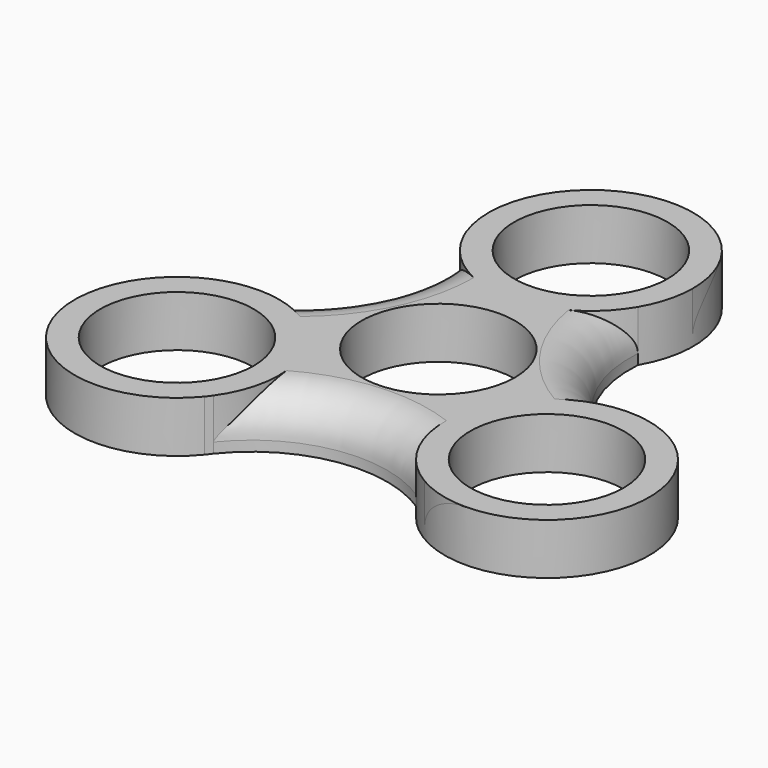
from build123d import *

# Parameters (mm, degrees)
F0_R         = 9.525
F1_DEPTH     = 6.35
F2_T4_ANGLE  = 171.8918539933
F2_S5_R      = 12.7
F2_T6_DEPTH  = 33
F2_S7_R      = 12.7
F2_T8_DEPTH  = 33
F2_T12_ANGLE = 171.8918539933
F2_S13_R     = 12.7
F2_T14_DEPTH = 34
F2_S15_R     = 12.7
F2_T16_DEPTH = 34
F2_T20_ANGLE = 171.8918539933
F2_S21_R     = 12.7
F2_T22_DEPTH = 33
F2_S23_R     = 12.7
F2_T24_DEPTH = 33


# Not quite as in the source:
# - a fillet or chamfer that OpenCascade refuses, or shapes differently, is made with other operations: its cross-section is extruded or revolved along the edge and cut away or added


with BuildPart() as f1:
    # F0 (on Top) → F1 (new body)
    with BuildSketch(Plane.XY):
        with BuildLine():
            ThreePointArc((-16.9151689036, 34.8937534074), (-16.926787396, 22.6379285555), (-25.2467054302, 13.6387985033))
            ThreePointArc((-25.2467054302, 13.6387985033), (-36.7990792752, -4.4780457484), (-15.4716495202, -7.0892001179))
            ThreePointArc((-15.4716495202, -7.0892001179), (-15.2019637006, -6.723178945), (-14.922490674, -6.3645750302))
            ThreePointArc((-14.922490674, -6.3645750302), (-4.3028257617, -0.2467245138), (7.6506084925, -2.9524198627))
            ThreePointArc((7.6506084925, -2.9524198627), (29.1164427734, -3.8986469606), (20.7140539132, 15.8770261894))
            ThreePointArc((20.7140539132, 15.8770261894), (20.2622273693, 15.9275703737), (19.8119307558, 15.9902991571))
            ThreePointArc((19.8119307558, 15.9902991571), (9.2038843359, 22.1282734926), (5.5703681159, 33.8330988937))
            ThreePointArc((5.5703681159, 33.8330988937), (-4.34309232, 52.8961702433), (-17.2681332147, 35.7316514628))
            ThreePointArc((-17.2681332147, 35.7316514628), (-17.0859924904, 35.3150861055), (-16.9151689036, 34.8937534074))
        make_face()
        with Locations((-25.31230589, 0.9389679304)):
            Circle(F0_R, mode=Mode.SUBTRACT)
        with Locations((-4.0085762739, 14.8398258448)):
            Circle(F0_R, mode=Mode.SUBTRACT)
        with Locations((18.6817846223, 3.3406837591)):
            Circle(F0_R, mode=Mode.SUBTRACT)
        with Locations((-5.3952075541, 40.2398258448)):
            Circle(F0_R, mode=Mode.SUBTRACT)
        with BuildLine():
            ThreePointArc((-14.922490674, -6.3645750302), (-15.2019637006, -6.723178945), (-15.4716495202, -7.0892001179))
            ThreePointArc((-15.4716495202, -7.0892001179), (-15.1905834316, -6.7318035089), (-14.922490674, -6.3645750302))
        make_face()
        with BuildLine():
            ThreePointArc((-17.2681332147, 35.7316514628), (-17.0991517164, 35.3095427854), (-16.9151689036, 34.8937534074))
            ThreePointArc((-16.9151689036, 34.8937534074), (-17.0859924904, 35.3150861055), (-17.2681332147, 35.7316514628))
        make_face()
        with BuildLine():
            ThreePointArc((19.8119307558, 15.9902991571), (20.2622273693, 15.9275703737), (20.7140539132, 15.8770261894))
            ThreePointArc((20.7140539132, 15.8770261894), (20.2640063262, 15.9417382578), (19.8119307558, 15.9902991571))
        make_face()
    extrude(amount=F1_DEPTH)

    # F2: fillet of radius 5.08 on 3 edges, made by hand


with BuildPart() as f2_tool2:
    # F2_s3 → F2_t4 (revolve)
    with BuildSketch(Plane(origin=(1.3219976545, -16.6427211425, 0), x_dir=(0, 0, 1), z_dir=(0.0791845597, -0.9968599729, 0))):
        with BuildLine():
            ThreePointArc((1.27, 19.9508919573), (4.8621024484, 21.4387895089), (6.35, 25.0308919573))
            Line((6.35, 25.0308919573), (6.35, 19.9508919573))
            Line((6.35, 19.9508919573), (1.27, 19.9508919573))
        make_face()
    revolve(axis=Axis((-1.7870715149, -16.8896868949, 6.35), (0, 0, -1)), revolution_arc=F2_T4_ANGLE)

    # F2_s5 → F2_t6 (cut, symmetric)
    with BuildSketch(Plane.XY.offset(2)):
        with Locations((-25.31230589, 0.9389679304)):
            Circle(F2_S5_R)
    extrude(amount=F2_T6_DEPTH, both=True, mode=Mode.SUBTRACT)

    # F2_s7 → F2_t8 (cut, symmetric)
    with BuildSketch(Plane.XY.offset(2)):
        with Locations((18.6817846223, 3.3406837591)):
            Circle(F2_S7_R)
    extrude(amount=F2_T8_DEPTH, both=True, mode=Mode.SUBTRACT)


with BuildPart() as f1_1:
    add(f1.part)

    # F2_t1: cut F2_tool2
    add(f2_tool2.part, mode=Mode.SUBTRACT)


with BuildPart() as f2_tool10:
    # F2_s11 → F2_t12 (revolve)
    with BuildSketch(Plane(origin=(30.4099792651, 20.9327995218, 0), x_dir=(0, 0, 1), z_dir=(0.8237137807, 0.5670058267, 0))):
        with BuildLine():
            ThreePointArc((1.27, 2.6333326422), (4.8621024484, 4.1212301938), (6.35, 7.7133326422))
            Line((6.35, 7.7133326422), (6.35, 2.6333326422))
            Line((6.35, 2.6333326422), (1.27, 2.6333326422))
        make_face()
    revolve(axis=Axis((22.3592354288, 32.6284617706, 6.35), (0, 0, -1)), revolution_arc=F2_T12_ANGLE)

    # F2_s13 → F2_t14 (cut, symmetric)
    with BuildSketch(Plane.XY.offset(2)):
        with Locations((18.6817846223, 3.3406837591)):
            Circle(F2_S13_R)
    extrude(amount=F2_T14_DEPTH, both=True, mode=Mode.SUBTRACT)

    # F2_s15 → F2_t16 (cut, symmetric)
    with BuildSketch(Plane.XY.offset(2)):
        with Locations((-5.3952075541, 40.2398258448)):
            Circle(F2_S15_R)
    extrude(amount=F2_T16_DEPTH, both=True, mode=Mode.SUBTRACT)


with BuildPart() as f1_2:
    add(f1_1.part)

    # F2_t9: cut F2_tool10
    add(f2_tool10.part, mode=Mode.SUBTRACT)


with BuildPart() as f2_tool18:
    # F2_s19 → F2_t20 (revolve)
    with BuildSketch(Plane(origin=(-37.7448413305, 17.9696603878, 0), x_dir=(0, 0, 1), z_dir=(-0.9028983404, 0.4298541461, 0))):
        with BuildLine():
            ThreePointArc((1.27, 28.8057387926), (4.8621024484, 30.2936363442), (6.35, 33.8857387926))
            Line((6.35, 33.8857387926), (6.35, 28.8057387926))
            Line((6.35, 28.8057387926), (1.27, 28.8057387926))
        make_face()
    revolve(axis=Axis((-32.5978927357, 28.7807026587, 6.35), (0, 0, -1)), revolution_arc=F2_T20_ANGLE)

    # F2_s21 → F2_t22 (cut, symmetric)
    with BuildSketch(Plane.XY.offset(2)):
        with Locations((-25.31230589, 0.9389679304)):
            Circle(F2_S21_R)
    extrude(amount=F2_T22_DEPTH, both=True, mode=Mode.SUBTRACT)

    # F2_s23 → F2_t24 (cut, symmetric)
    with BuildSketch(Plane.XY.offset(2)):
        with Locations((-5.3952075541, 40.2398258448)):
            Circle(F2_S23_R)
    extrude(amount=F2_T24_DEPTH, both=True, mode=Mode.SUBTRACT)


with BuildPart() as f1_3:
    add(f1_2.part)

    # F2_t17: cut F2_tool18
    add(f2_tool18.part, mode=Mode.SUBTRACT)


solid = f1_3.part
